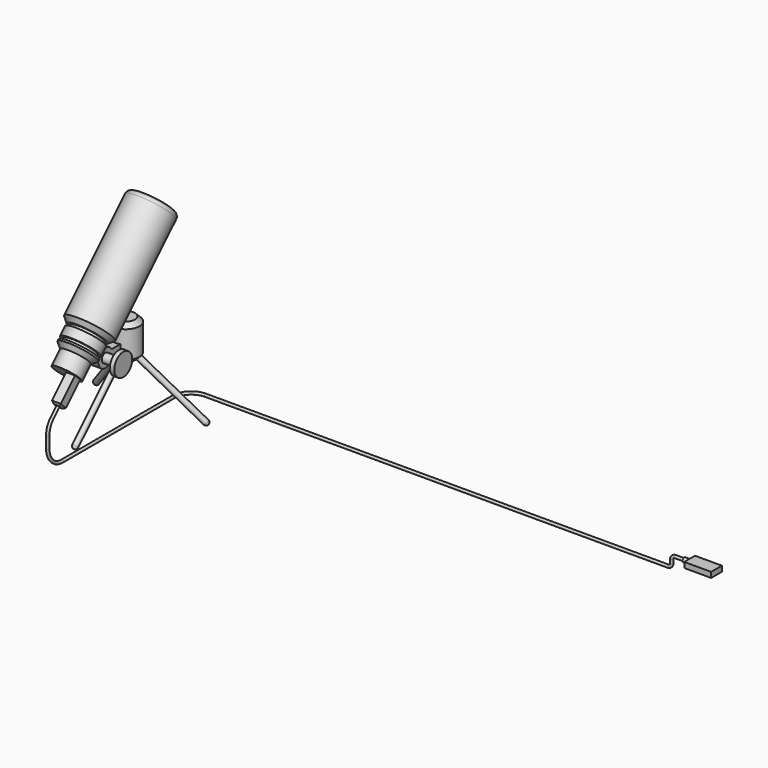
from build123d import *

# Parameters (mm, degrees)
F0_R      = 15
F1_DEPTH  = 40
F2_SIZE   = 5
F12_W     = 10
F12_H     = 10
F13_DEPTH = 30
F15_DEPTH = 5
F16_R     = 20
F17_DEPTH = 10
F20_R     = 5
F21_SIZE  = 4.99999
F22_R     = 5
F23_DEPTH = 15
F24_R     = 12.5
F25_DEPTH = 5
F26_W     = 10
F26_H     = 10
F27_DEPTH = 30
F28_SIZE  = 2
F30_R     = 1.5
F32_R     = 1.5
F36_R     = 1.5
F40_W     = 15
F40_H     = 6
F41_DEPTH = 30
F42_R     = 2.5
F43_DEPTH = 6


# Not quite as in the source:
# - a fillet or chamfer is up to 0.001 mm smaller than in the source, because OpenCascade refuses the exact size


with BuildPart() as f1:
    # F0 (on Top) → F1 (new body)
    with BuildSketch(Plane.XY):
        Circle(F0_R)
    extrude(amount=F1_DEPTH)

    # F2
    f2_edges = [f1.edges().sort_by_distance(p)[0] for p in [
        (-15, 0, 0),
        (-15, 0, 40),
    ]]
    chamfer(f2_edges, length=F2_SIZE)

    # F3 (on Right) → F4 (revolve)
    with BuildSketch(Plane.YZ):
        with BuildLine():
            Line((-2.1213203436, 14.1213203436), (-72.8319984622, -56.5893577751))
            ThreePointArc((-72.8319984622, -56.5893577751), (-73.7106781187, -58.7106781187), (-72.8319984622, -60.8319984622))
            Line((-72.8319984622, -60.8319984622), (0, 12))
            Line((0, 12), (-2.1213203436, 14.1213203436))
        make_face()
    revolve(axis=Axis((0, -36.4159992311, -24.4159992311), (0, 0.7071067812, 0.7071067812)))

    # F7 (on line) → F8 (revolve)
    with BuildSketch(Plane(origin=(0, 0, 0), x_dir=(0.8660254038, 0.5, 0), z_dir=(0.5, -0.8660254038, 0))):
        with BuildLine():
            Line((2.0230960578, 14.2195446293), (0, 12))
            Line((0, 12), (72.7337741765, -60.7337741765))
            ThreePointArc((72.7337741765, -60.7337741765), (73.6124538329, -58.6124538329), (72.7337741765, -56.4911334894))
            Line((72.7337741765, -56.4911334894), (2.0230960578, 14.2195446293))
        make_face()
    revolve(axis=Axis((31.494648075, 18.1834435441, -24.3668870882), (0.6123724357, 0.3535533906, -0.7071067812)))

    # F10 (on face) → F11 (revolve)
    with BuildSketch(Plane(origin=(0, 0, 0), x_dir=(0.8660254038, -0.5, 0), z_dir=(-0.5, -0.8660254038, 0))):
        with BuildLine():
            Line((-72.8869811403, -60.8869811403), (0, 12))
            Line((0, 12), (-2.1763030217, 14.0663376655))
            Line((-2.1763030217, 14.0663376655), (-72.8869811403, -56.6443404532))
            ThreePointArc((-72.8869811403, -56.6443404532), (-73.7656607968, -58.7656607968), (-72.8869811403, -60.8869811403))
        make_face()
    revolve(axis=Axis((-31.5609886363, 18.2217452851, -24.4434905702), (-0.6123724357, 0.3535533906, -0.7071067812)))

    # F12 (on Front) → F13 (join)
    with BuildSketch(Plane.XZ):
        with Locations((0, 15)):
            Rectangle(F12_W, F12_H)
    extrude(amount=F13_DEPTH)

    # F14 (on Right) → F15 (join, symmetric)
    with BuildSketch(Plane.YZ):
        with BuildLine():
            ThreePointArc((-44.6592582629, 17.588190451), (-36.3052619222, 5.0855513863), (-25, 15))
            ThreePointArc((-25, 15), (-28.9123857099, 22.9335334029), (-37.588190451, 24.6592582629))
            Line((-37.588190451, 24.6592582629), (-31.4644660941, 18.5355339059))
            Line((-31.4644660941, 18.5355339059), (-35, 15))
            Line((-35, 15), (-38.5355339059, 11.4644660941))
            Line((-38.5355339059, 11.4644660941), (-44.6592582629, 17.588190451))
        make_face()
        with BuildLine():
            Line((-31.4644660941, 18.5355339059), (-37.588190451, 24.6592582629))
            ThreePointArc((-37.588190451, 24.6592582629), (-42.0710678119, 22.0710678119), (-44.6592582629, 17.588190451))
            Line((-44.6592582629, 17.588190451), (-38.5355339059, 11.4644660941))
            Line((-38.5355339059, 11.4644660941), (-35, 15))
            Line((-35, 15), (-31.4644660941, 18.5355339059))
        make_face()
        with BuildLine():
            ThreePointArc((-44.6592582629, 17.588190451), (-42.0710678119, 22.0710678119), (-37.588190451, 24.6592582629))
            Line((-37.588190451, 24.6592582629), (-45.6066017178, 32.6776695297))
            Line((-45.6066017178, 32.6776695297), (-52.6776695297, 25.6066017178))
            Line((-52.6776695297, 25.6066017178), (-44.6592582629, 17.588190451))
        make_face()
    extrude(amount=F15_DEPTH, both=True)

    # F16 (on face) → F17 (join)
    with BuildSketch(Plane(origin=(0, -6.4644660941, -6.4644660941), x_dir=(1, 0, 0), z_dir=(0, 0.7071067812, 0.7071067812))):
        with Locations((0, -70.3553390593)):
            Circle(F16_R)
    extrude(amount=-F17_DEPTH)

    # F18 (on Right) → F19 (revolve)
    with BuildSketch(Plane.YZ):
        Polygon((-89.4472221514, 24.1923881554), (-82.3761543395, 17.1213203436), (37.8319984622, 137.3294731453), (20.1543289326, 155.0071426749), (-71.7695526217, 63.0832611207), (-66.1126983722, 57.4264068712), (-77.4264068712, 46.1126983722), (-79.5477272148, 48.2340187158), (-84.4974746831, 43.2842712475), (-80.9619407771, 39.7487373415), (-92.9827560573, 27.7279220614), align=None)
    revolve(axis=Axis((0, -22.2720779386, 77.2253967444), (0, 0.7071067812, 0.7071067812)))

    # F20
    f20_edges = [f1.edges().sort_by_distance(p)[0] for p in [
        (0, 55.509668, 119.651804),
    ]]
    fillet(f20_edges, radius=F20_R)

    # F21 (size 5 in the source; OpenCascade refuses exactly that, so slightly less here)
    f21_edges = [f1.edges().sort_by_distance(p)[0] for p in [
        (0, -36.414214, 27.727922),
        (0, -56.213203, 15),
    ]]
    chamfer(f21_edges, length=F21_SIZE)

    # F22 (on face) → F23 (join)
    with BuildSketch(Plane.YZ.offset(5)):
        with Locations((-35, 15)):
            Circle(F22_R)
    extrude(amount=F23_DEPTH)

    # F24 (on face) → F25 (join)
    with BuildSketch(Plane.YZ.offset(20)):
        with Locations((-35, 15)):
            Circle(F24_R)
    extrude(amount=F25_DEPTH)

    # F26 (on face) → F27 (join)
    with BuildSketch(Plane(origin=(0, -32.627416998, -32.627416998), x_dir=(1, 0, 0), z_dir=(0, -0.7071067812, -0.7071067812))):
        with Locations((7, 70.3553390593)):
            Rectangle(F26_W, F26_H)
    extrude(amount=F27_DEPTH)

    # F28
    f28_edges = [f1.edges().sort_by_distance(p)[0] for p in [
        (2, -103.589358, -4.091883),
        (7, -100.053824, -7.627417),
        (12, -103.589358, -4.091883),
        (7, -107.124892, -0.556349),
    ]]
    chamfer(f28_edges, length=F28_SIZE)

    # F31: sweep along a path in F29
    with BuildLine(Plane.YZ) as f31_path:
        Line((-103.5893577751, -4.091883092), (-111.8736290226, -12.3761543395))
        ThreePointArc((-111.8736290226, -12.3761543395), (-116.2090840491, -18.8646213159), (-117.7314933988, -26.5182899632))
        Line((-117.7314933988, -26.5182899632), (-117.7314933988, -40.2340187158))
        ThreePointArc((-117.7314933988, -40.2340187158), (-111.8736290226, -54.3761543395), (-97.7314933988, -60.2340187158))
        Line((-97.7314933988, -60.2340187158), (52.2685066012, -60.2340187158))
    # F30 (on face) → F31 (sweep)
    with BuildSketch(Plane(origin=(0, -53.8406204336, -53.8406204336), x_dir=(1, 0, 0), z_dir=(0, -0.7071067812, -0.7071067812))):
        with Locations((7, 70.3553390593)):
            Circle(F30_R)
    sweep(path=f31_path.line)

    # F35: sweep along a path in F34
    with BuildLine(Plane.XY.offset(-60.2340187158)) as f35_path:
        Line((527, 77.2685066012), (27, 77.2685066012))
        ThreePointArc((27, 77.2685066012), (12.8578643763, 71.4106422249), (7, 57.2685066012))
        Line((7, 57.2685066012), (7, 52.2685066012))
    # F32 (on face) → F35 (sweep)
    with BuildSketch(Plane(origin=(0, 52.2685066012, 0), x_dir=(-1, 0, 0), z_dir=(0, 1, 0))):
        with Locations((-7, -60.2340187158)):
            Circle(F32_R)
    sweep(path=f35_path.line)

    # F39: sweep along a path in F38
    with BuildLine(Plane(origin=(0, 77.2685066012, 0), x_dir=(-1, 0, 0), z_dir=(0, 1, 0))) as f39_path:
        Line((-527, -60.2340187158), (-543, -60.2340187158))
        ThreePointArc((-543, -60.2340187158), (-545.8284271247, -59.0624458405), (-547, -56.2340187158))
        Line((-547, -56.2340187158), (-547, -52.2340187158))
        ThreePointArc((-547, -52.2340187158), (-548.1715728753, -49.405591591), (-551, -48.2340187158))
        Line((-551, -48.2340187158), (-567, -48.2340187158))
    # F36 (on face) → F39 (sweep)
    with BuildSketch(Plane.YZ.offset(527)):
        with Locations((77.2685066012, -60.2340187158)):
            Circle(F36_R)
    sweep(path=f39_path.line)

    # F40 (on face) → F41 (join)
    with BuildSketch(Plane.YZ.offset(567)):
        with Locations((77.2685066012, -48.2340187158)):
            Rectangle(F40_W, F40_H)
    extrude(amount=F41_DEPTH)

    # F42 (on face) → F43 (join)
    with BuildSketch(Plane(origin=(567, 0, 0), x_dir=(0, -1, 0), z_dir=(-1, 0, 0))):
        with Locations((-77.2685066012, -48.2340187158)):
            Circle(F42_R)
    extrude(amount=F43_DEPTH)


solid = f1.part
